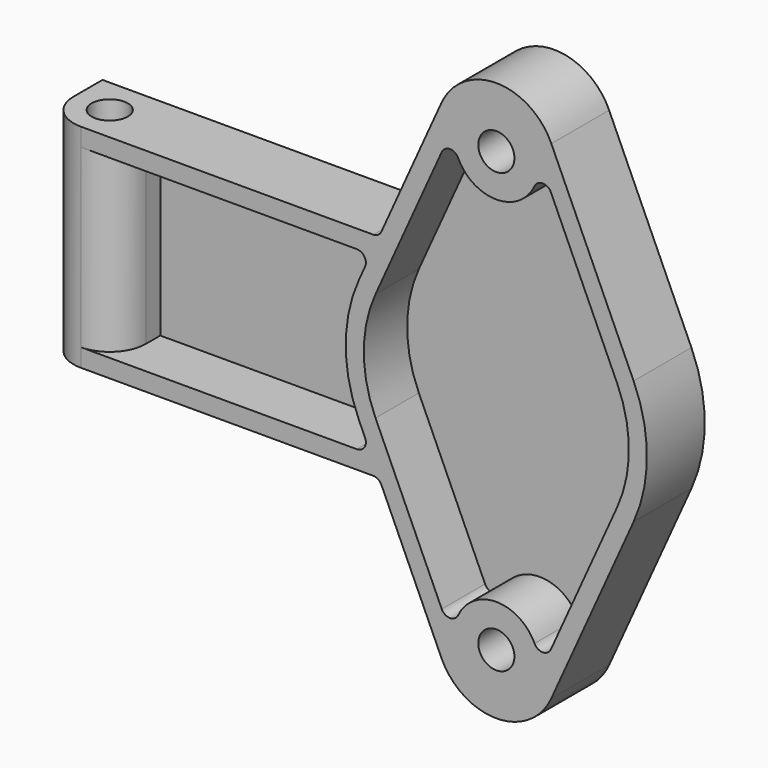
from build123d import *

# Parameters (mm, degrees)
F0_R     = 2
F1_DEPTH = 8
F2_DEPTH = 2
F3_R     = 1
F5_D     = 4
F6_R     = 3.99999


# Not quite as in the source:
# - a fillet or chamfer is up to 0.001 mm smaller than in the source, because OpenCascade refuses the exact size
# - a feature names something its author has since deleted; it is built from what else it names


with BuildPart() as f1:
    # F0 (on Front) → F1 (new body)
    with BuildSketch(Plane.XZ):
        with BuildLine():
            Line((15.1970139668, 6.8636525628), (6.0880650012, 27.0320429916))
            ThreePointArc((6.0880650012, 27.0320429916), (0, 30.9626), (-6.0880650012, 27.0320429916))
            Line((-6.0880650012, 27.0320429916), (-12.9901204821, 11.75))
            Line((-12.9901204821, 11.75), (-13.8934101123, 9.75))
            Line((-13.8934101123, 9.75), (-15.1970139668, 6.8636525628))
            ThreePointArc((-15.1970139668, 6.8636525628), (-16.6751, 0), (-15.1970139668, -6.8636525628))
            Line((-15.1970139668, -6.8636525628), (-13.8934101123, -9.75))
            Line((-13.8934101123, -9.75), (-12.9901204821, -11.75))
            Line((-12.9901204821, -11.75), (-6.0880650012, -27.0320429916))
            ThreePointArc((-6.0880650012, -27.0320429916), (0, -30.9626), (6.0880650012, -27.0320429916))
            Line((6.0880650012, -27.0320429916), (15.1970139668, -6.8636525628))
            ThreePointArc((15.1970139668, -6.8636525628), (16.6751, 0), (15.1970139668, 6.8636525628))
        make_face()
        with Locations((0, -24.2824)):
            Circle(F0_R, mode=Mode.SUBTRACT)
        with BuildLine():
            Line((-13.3742945868, 6.0404308054), (-6.0462846285, 22.2655920687))
            ThreePointArc((-6.0462846285, 22.2655920687), (-5.1436901116, 22.8539427752), (-4.2309206889, 22.2815046593))
            ThreePointArc((-4.2309206889, 22.2815046593), (0, 19.6022), (4.2309206889, 22.2815046593))
            ThreePointArc((4.2309206889, 22.2815046593), (5.1436901116, 22.8539427752), (6.0462846285, 22.2655920687))
            Line((6.0462846285, 22.2655920687), (13.3742945868, 6.0404308054))
            ThreePointArc((13.3742945868, 6.0404308054), (14.6751, 0), (13.3742945868, -6.0404308054))
            Line((13.3742945868, -6.0404308054), (6.0462846285, -22.2655920687))
            ThreePointArc((6.0462846285, -22.2655920687), (5.1436901116, -22.8539427752), (4.2309206889, -22.2815046593))
            ThreePointArc((4.2309206889, -22.2815046593), (0, -19.6022), (-4.2309206889, -22.2815046593))
            ThreePointArc((-4.2309206889, -22.2815046593), (-5.1436901116, -22.8539427752), (-6.0462846285, -22.2655920687))
            Line((-6.0462846285, -22.2655920687), (-13.3742945868, -6.0404308054))
            ThreePointArc((-13.3742945868, -6.0404308054), (-14.6751, 0), (-13.3742945868, 6.0404308054))
        make_face(mode=Mode.SUBTRACT)
        with Locations((0, 24.2824)):
            Circle(F0_R, mode=Mode.SUBTRACT)
        Polygon((-13.8934101123, 9.75), (-12.9901204821, 11.75), (-50, 11.75), (-50, -11.75), (-12.9901204821, -11.75), (-13.8934101123, -9.75), (-42, -9.75), (-42, 9.75), align=None)
    extrude(amount=F1_DEPTH)

    # F0 (on Front) → F2 (join)
    with BuildSketch(Plane.XZ):
        with BuildLine():
            Line((15.1970139668, 6.8636525628), (6.0880650012, 27.0320429916))
            ThreePointArc((6.0880650012, 27.0320429916), (0, 30.9626), (-6.0880650012, 27.0320429916))
            Line((-6.0880650012, 27.0320429916), (-12.9901204821, 11.75))
            Line((-12.9901204821, 11.75), (-13.8934101123, 9.75))
            Line((-13.8934101123, 9.75), (-15.1970139668, 6.8636525628))
            ThreePointArc((-15.1970139668, 6.8636525628), (-16.6751, 0), (-15.1970139668, -6.8636525628))
            Line((-15.1970139668, -6.8636525628), (-13.8934101123, -9.75))
            Line((-13.8934101123, -9.75), (-12.9901204821, -11.75))
            Line((-12.9901204821, -11.75), (-6.0880650012, -27.0320429916))
            ThreePointArc((-6.0880650012, -27.0320429916), (0, -30.9626), (6.0880650012, -27.0320429916))
            Line((6.0880650012, -27.0320429916), (15.1970139668, -6.8636525628))
            ThreePointArc((15.1970139668, -6.8636525628), (16.6751, 0), (15.1970139668, 6.8636525628))
        make_face()
        with Locations((0, -24.2824)):
            Circle(F0_R, mode=Mode.SUBTRACT)
        with BuildLine():
            Line((-13.3742945868, 6.0404308054), (-6.0462846285, 22.2655920687))
            ThreePointArc((-6.0462846285, 22.2655920687), (-5.1436901116, 22.8539427752), (-4.2309206889, 22.2815046593))
            ThreePointArc((-4.2309206889, 22.2815046593), (0, 19.6022), (4.2309206889, 22.2815046593))
            ThreePointArc((4.2309206889, 22.2815046593), (5.1436901116, 22.8539427752), (6.0462846285, 22.2655920687))
            Line((6.0462846285, 22.2655920687), (13.3742945868, 6.0404308054))
            ThreePointArc((13.3742945868, 6.0404308054), (14.6751, 0), (13.3742945868, -6.0404308054))
            Line((13.3742945868, -6.0404308054), (6.0462846285, -22.2655920687))
            ThreePointArc((6.0462846285, -22.2655920687), (5.1436901116, -22.8539427752), (4.2309206889, -22.2815046593))
            ThreePointArc((4.2309206889, -22.2815046593), (0, -19.6022), (-4.2309206889, -22.2815046593))
            ThreePointArc((-4.2309206889, -22.2815046593), (-5.1436901116, -22.8539427752), (-6.0462846285, -22.2655920687))
            Line((-6.0462846285, -22.2655920687), (-13.3742945868, -6.0404308054))
            ThreePointArc((-13.3742945868, -6.0404308054), (-14.6751, 0), (-13.3742945868, 6.0404308054))
        make_face(mode=Mode.SUBTRACT)
        with Locations((0, 24.2824)):
            Circle(F0_R, mode=Mode.SUBTRACT)
        with BuildLine():
            ThreePointArc((-4.2309206889, 22.2815046593), (-5.1436901116, 22.8539427752), (-6.0462846285, 22.2655920687))
            Line((-6.0462846285, 22.2655920687), (-13.3742945868, 6.0404308054))
            ThreePointArc((-13.3742945868, 6.0404308054), (-14.6751, 0), (-13.3742945868, -6.0404308054))
            Line((-13.3742945868, -6.0404308054), (-6.0462846285, -22.2655920687))
            ThreePointArc((-6.0462846285, -22.2655920687), (-5.1436901116, -22.8539427752), (-4.2309206889, -22.2815046593))
            ThreePointArc((-4.2309206889, -22.2815046593), (0, -19.6022), (4.2309206889, -22.2815046593))
            ThreePointArc((4.2309206889, -22.2815046593), (5.1436901116, -22.8539427752), (6.0462846285, -22.2655920687))
            Line((6.0462846285, -22.2655920687), (13.3742945868, -6.0404308054))
            ThreePointArc((13.3742945868, -6.0404308054), (14.6751, 0), (13.3742945868, 6.0404308054))
            Line((13.3742945868, 6.0404308054), (6.0462846285, 22.2655920687))
            ThreePointArc((6.0462846285, 22.2655920687), (5.1436901116, 22.8539427752), (4.2309206889, 22.2815046593))
            ThreePointArc((4.2309206889, 22.2815046593), (0, 19.6022), (-4.2309206889, 22.2815046593))
        make_face()
        with BuildLine():
            Line((-15.1970139668, 6.8636525628), (-13.8934101123, 9.75))
            Line((-13.8934101123, 9.75), (-42, 9.75))
            Line((-42, 9.75), (-42, -9.75))
            Line((-42, -9.75), (-13.8934101123, -9.75))
            Line((-13.8934101123, -9.75), (-15.1970139668, -6.8636525628))
            ThreePointArc((-15.1970139668, -6.8636525628), (-16.6751, 0), (-15.1970139668, 6.8636525628))
        make_face()
    extrude(amount=F2_DEPTH)

    # F3
    f3_edges = [f1.edges().sort_by_distance(p)[0] for p in [
        (-13.89341, -5, -9.75),
        (-12.99012, -4, -11.75),
        (-13.89341, -5, 9.75),
        (-12.99012, -4, 11.75),
    ]]
    fillet(f3_edges, radius=F3_R)

    # F5 (through all)
    with Locations(Plane.XY.offset(11.75)):
        with Locations((-46, -4)):
            Hole(F5_D / 2)

    # F6 (radius 4 in the source; OpenCascade refuses exactly that, so slightly less here)
    f6_edges = [f1.edges().sort_by_distance(p)[0] for p in [
        (-50, -8, 0),
        (-42, -8, 0),
    ]]
    fillet(f6_edges, radius=F6_R)


solid = f1.part
